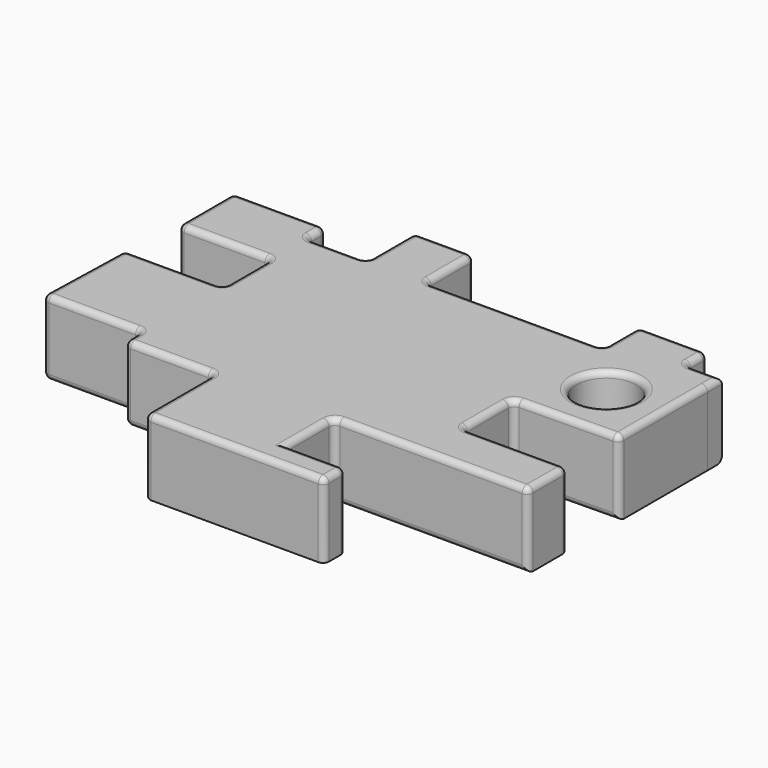
from build123d import *

# Parameters (mm, degrees)
F0_W     = 20
F0_H     = 20
F0_H_2   = 9
F0_R     = 10
F0_W_2   = 12
F0_H_3   = 6
F1_DEPTH = 25
F2_F1_R  = 2
F2_F2_R  = 2


# Not quite as in the source:
# - a feature names something its author has since deleted; it is built from what else it names


with BuildPart() as f1:
    # F0 (on Top) → F1 (new body)
    with BuildSketch(Plane.XY):
        Polygon((34.8936983969, 37.4976433316), (-24.1063016031, 37.4976433316), (-44.1063016031, 37.4976433316), (-44.1063016031, 2.4976433316), (-45.1040744059, -37.48991035), (-35.1040744059, -37.48991035), (4.8959255941, -37.48991035), (34.8959255941, -37.48991035), (69.8936983969, -37.48991035), (69.8936983969, -20.9999998819), (34.8936983969, -20.9999998819), (34.8959255941, 0), align=None)
        Polygon((-44.1063016031, 2.4976433316), (-44.1063016031, 37.4976433316), (-64.1063016031, 37.4976433316), (-64.1063016031, 22.4976433316), (-64.1063016031, 2.4976433316), align=None)
        Polygon((-64.1063016031, 22.4976433316), (-64.1063016031, 37.4976433316), (-64.1063016031, 45.4976433316), (-95.1063016031, 45.4976433316), (-95.1063016031, 22.4976433316), align=None)
        with Locations((-34.1063016031, 47.4976433316)):
            Rectangle(F0_W, F0_H)
        Polygon((-45.1040744059, -37.48991035), (-44.1063016031, 2.4976433316), (-64.1063016031, 2.4976433316), (-65.0125588003, -30.48991035), (-65.0125588003, -37.48991035), align=None)
        Polygon((-65.0125588003, -30.48991035), (-64.1063016031, 2.4976433316), (-97.1063016031, 2.4976433316), (-98.0125588003, -30.48991035), align=None)
        Polygon((4.8959255941, -37.48991035), (-35.1040744059, -37.48991035), (-35.1040744059, -66.48991035), (4.8959255941, -66.48991035), (4.8959255941, -57.48991035), align=None)
        with Locations((14.8959255941, -61.98991035)):
            Rectangle(F0_W, F0_H_2)
        Polygon((57.8936983969, 37.4976433316), (34.8936983969, 37.4976433316), (34.8959255941, 0), (69.8923875736, 0.4976433634), (69.8936983969, 37.4976433316), align=None)
        with Locations((50.4960529506, 19.4228515029)):
            Circle(F0_R, mode=Mode.SUBTRACT)
        Polygon((34.8936983969, 52.4976433316), (34.8936983969, 37.4976433316), (57.8936983969, 37.4976433316), (57.8936983969, 43.4976433316), (57.8936983969, 52.4976433316), align=None)
        with Locations((63.8936983969, 40.4976433316)):
            Rectangle(F0_W_2, F0_H_3)
    extrude(amount=F1_DEPTH)

    # F2: fillet of radius 2 on 86 edges, made by hand

    # F2_f1
    f2_f1_edges = [f1.edges().sort_by_distance(p)[0] for p in [
        (-64.1063016031, 2.4976433316, 12.5),
        (57.8936983969, 43.4976433316, 12.5),
        (34.8936983969, -20.9999998819, 12.5),
        (-35.1040744059, -37.48991035, 12.5),
        (-64.1063016031, 22.4976433316, 12.5),
        (4.8959255941, -37.48991035, 12.5),
        (34.8959255941, 0, 12.5),
        (34.8936983969, 37.4976433316, 12.5),
        (-24.1063016031, 37.4976433316, 12.5),
        (-44.1063016031, 37.4976433316, 12.5),
        (-64.1063016031, 37.4976433316, 12.5),
        (-65.0125588003, -30.48991035, 12.5),
    ]]
    fillet(f2_f1_edges, radius=F2_F1_R)

    # F2_f2
    f2_f2_edges = [f1.edges().sort_by_distance(p)[0] for p in [
        (-44.1063016031, 48.4976433316, 25),
        (-34.1063016031, 57.4976433316, 25),
        (-24.1063016031, 48.4976433316, 25),
        (5.3936983969, 37.4976433316, 25),
        (34.8936983969, 45.9976433316, 25),
        (46.3936983969, 52.4976433316, 25),
        (57.8936983969, 48.9976433316, 25),
        (64.8936983969, 43.4976433316, 25),
        (69.8936983969, 40.4976433316, 25),
        (53.3798336479, 0.2628378314, 25),
        (34.8948135152, -10.485670591, 25),
        (53.3938044596, -20.9999998819, 25),
        (69.8936983969, -29.2449551159, 25),
        (38.3948119955, -37.48991035, 25),
        (4.8959255941, -48.48991035, 25),
        (14.8959255941, -57.48991035, 25),
        (24.8959255941, -61.98991035, 25),
        (-5.1040744059, -66.48991035, 25),
        (-35.1040744059, -52.98991035, 25),
        (-51.0583166031, -37.48991035, 25),
        (-65.0125588003, -34.98991035, 25),
        (-82.5125588003, -30.48991035, 25),
        (-97.5594302017, -13.9961335092, 25),
        (-81.6063016031, 2.4976433316, 25),
        (-64.1063016031, 12.4976433316, 25),
        (-80.6063016031, 22.4976433316, 25),
        (-95.1063016031, 33.9976433316, 25),
        (-79.6063016031, 45.4976433316, 25),
        (-64.1063016031, 42.4976433316, 25),
        (-54.1063016031, 37.4976433316, 25),
        (69.8930429853, 18.9976433475, 25),
        (-34.1063016031, 57.4976433316, 0),
        (-24.1063016031, 48.4976433316, 0),
        (5.3936983969, 37.4976433316, 0),
        (46.3936983969, 52.4976433316, 0),
        (34.8936983969, 45.9976433316, 0),
        (57.8936983969, 48.9976433316, 0),
        (64.8936983969, 43.4976433316, 0),
        (-44.1063016031, 48.4976433316, 0),
        (-54.1063016031, 37.4976433316, 0),
        (-79.6063016031, 45.4976433316, 0),
        (-95.1063016031, 33.9976433316, 0),
        (-80.6063016031, 22.4976433316, 0),
        (-64.1063016031, 12.4976433316, 0),
        (-81.6063016031, 2.4976433316, 0),
        (-98.0125588003, -30.48991035, 12.5),
        (4.8959255941, -48.48991035, 0),
        (14.8959255941, -57.48991035, 0),
        (38.3948119955, -37.48991035, 0),
        (53.3938044596, -20.9999998819, 0),
        (34.8948135152, -10.485670591, 0),
        (53.3798336479, 0.2628378314, 0),
        (-24.1063016031, 57.4976433316, 12.5),
        (-44.1063016031, 57.4976433316, 12.5),
        (-64.1063016031, 45.4976433316, 12.5),
        (-95.1063016031, 45.4976433316, 12.5),
        (57.8936983969, 52.4976433316, 12.5),
        (34.8936983969, 52.4976433316, 12.5),
        (-95.1063016031, 22.4976433316, 12.5),
        (-97.1063016031, 2.4976433316, 12.5),
        (-82.5125588003, -30.48991035, 0),
        (-65.0125588003, -34.98991035, 0),
        (-51.0583166031, -37.48991035, 0),
        (-65.0125588003, -37.48991035, 12.5),
        (-35.1040744059, -52.98991035, 0),
        (69.8923875736, 0.4976433634, 12.5),
        (24.8959255941, -57.48991035, 12.5),
        (24.8959255941, -66.48991035, 12.5),
        (69.8936983969, -37.48991035, 12.5),
        (69.8936983969, -20.9999998819, 12.5),
        (-35.1040744059, -66.48991035, 12.5),
        (-97.5594302017, -13.9961335092, 0),
        (40.4960529506, 19.4228515029, 0),
        (40.4960529506, 19.4228515029, 25),
        (-35.6898608435, -38.0756967876, 0),
        (-65.598345238, -31.0756967876, 0),
        (35.4715589556, -0.5675663509, 0),
        (35.4796219682, -20.4141384487, 0),
        (5.4817120317, -38.0756967876, 0),
        (-64.6920880407, 3.0834297692, 0),
        (-64.6920880407, 21.9118568939, 0),
        (-44.6920880407, 38.0834297692, 0),
        (-63.5205151654, 38.0834297692, 0),
        (58.4794848346, 44.0834297692, 0),
        (34.3079119593, 38.0834297692, 0),
        (-23.5205151654, 38.0834297692, 0),
        (-44.6920880407, 38.0834297692, 25),
        (-63.5205151654, 38.0834297692, 25),
        (-64.6920880407, 21.9118568939, 25),
        (-64.6920880407, 3.0834297692, 25),
        (-65.598345238, -31.0756967876, 25),
        (-35.6898608435, -38.0756967876, 25),
        (5.4817120317, -38.0756967876, 25),
        (35.4796219682, -20.4141384487, 25),
        (35.4715589556, -0.5675663509, 25),
        (58.4794848346, 44.0834297692, 25),
        (34.3079119593, 38.0834297692, 25),
        (-23.5205151654, 38.0834297692, 25),
    ]]
    fillet(f2_f2_edges, radius=F2_F2_R)


solid = f1.part
